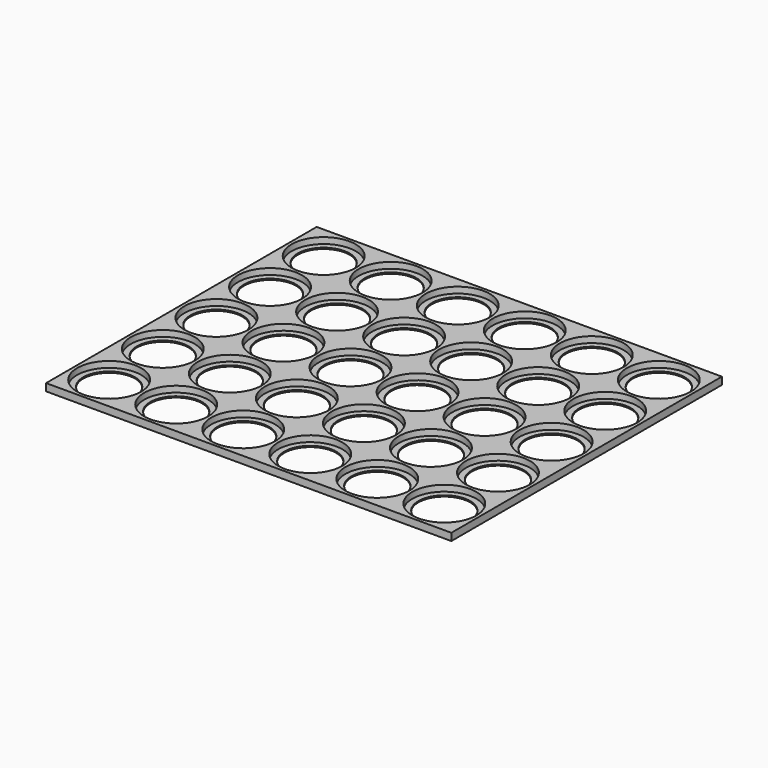
from build123d import *

# Parameters (mm, degrees)
F1_W      = 133
F1_H      = 111
F1_R      = 10.5
F2_DEPTH  = 2
F2_FACE_W = 133
F2_FACE_H = 111
F2_FACE_R = 10.5
F3_DEPTH  = 0.4
F4_D      = 17


# Not quite as in the source:
# - a feature of the source that left no trace in its solid (it failed there, or was rolled back) is left out


with BuildPart() as f2:
    # F1 (on Top) → F2 (new body)
    with BuildSketch(Plane.XY):
        with Locations((55, 44)):
            Rectangle(F1_W, F1_H)
        Circle(F1_R, mode=Mode.SUBTRACT)
        with Locations((22, 0)):
            Circle(F1_R, mode=Mode.SUBTRACT)
        with Locations((44, 0)):
            Circle(F1_R, mode=Mode.SUBTRACT)
        with Locations((0, 22)):
            Circle(F1_R, mode=Mode.SUBTRACT)
        with Locations((22, 22)):
            Circle(F1_R, mode=Mode.SUBTRACT)
        with Locations((44, 22)):
            Circle(F1_R, mode=Mode.SUBTRACT)
        with Locations((66, 0)):
            Circle(F1_R, mode=Mode.SUBTRACT)
        with Locations((88, 0)):
            Circle(F1_R, mode=Mode.SUBTRACT)
        with Locations((110, 0)):
            Circle(F1_R, mode=Mode.SUBTRACT)
        with Locations((66, 22)):
            Circle(F1_R, mode=Mode.SUBTRACT)
        with Locations((88, 22)):
            Circle(F1_R, mode=Mode.SUBTRACT)
        with Locations((110, 22)):
            Circle(F1_R, mode=Mode.SUBTRACT)
        with Locations((0, 44)):
            Circle(F1_R, mode=Mode.SUBTRACT)
        with Locations((0, 66)):
            Circle(F1_R, mode=Mode.SUBTRACT)
        with Locations((22, 44)):
            Circle(F1_R, mode=Mode.SUBTRACT)
        with Locations((44, 44)):
            Circle(F1_R, mode=Mode.SUBTRACT)
        with Locations((22, 66)):
            Circle(F1_R, mode=Mode.SUBTRACT)
        with Locations((44, 66)):
            Circle(F1_R, mode=Mode.SUBTRACT)
        with Locations((0, 88)):
            Circle(F1_R, mode=Mode.SUBTRACT)
        with Locations((22, 88)):
            Circle(F1_R, mode=Mode.SUBTRACT)
        with Locations((44, 88)):
            Circle(F1_R, mode=Mode.SUBTRACT)
        with Locations((66, 44)):
            Circle(F1_R, mode=Mode.SUBTRACT)
        with Locations((88, 44)):
            Circle(F1_R, mode=Mode.SUBTRACT)
        with Locations((66, 66)):
            Circle(F1_R, mode=Mode.SUBTRACT)
        with Locations((88, 66)):
            Circle(F1_R, mode=Mode.SUBTRACT)
        with Locations((110, 44)):
            Circle(F1_R, mode=Mode.SUBTRACT)
        with Locations((110, 66)):
            Circle(F1_R, mode=Mode.SUBTRACT)
        with Locations((66, 88)):
            Circle(F1_R, mode=Mode.SUBTRACT)
        with Locations((88, 88)):
            Circle(F1_R, mode=Mode.SUBTRACT)
        with Locations((110, 88)):
            Circle(F1_R, mode=Mode.SUBTRACT)
    extrude(amount=F2_DEPTH)

    # F2_face (on face) + F1 (on Top) → F3 (join)
    with BuildSketch(Plane(origin=(55, 44, 2), x_dir=(1, 0, 0), z_dir=(0, 0, 1))):
        Rectangle(F2_FACE_W, F2_FACE_H)
        with Locations((-55, -44)):
            Circle(F2_FACE_R, mode=Mode.SUBTRACT)
        with Locations((-33, -44)):
            Circle(F2_FACE_R, mode=Mode.SUBTRACT)
        with Locations((-11, -44)):
            Circle(F2_FACE_R, mode=Mode.SUBTRACT)
        with Locations((-55, -22)):
            Circle(F2_FACE_R, mode=Mode.SUBTRACT)
        with Locations((-33, -22)):
            Circle(F2_FACE_R, mode=Mode.SUBTRACT)
        with Locations((-11, -22)):
            Circle(F2_FACE_R, mode=Mode.SUBTRACT)
        with Locations((11, -44)):
            Circle(F2_FACE_R, mode=Mode.SUBTRACT)
        with Locations((33, -44)):
            Circle(F2_FACE_R, mode=Mode.SUBTRACT)
        with Locations((55, -44)):
            Circle(F2_FACE_R, mode=Mode.SUBTRACT)
        with Locations((11, -22)):
            Circle(F2_FACE_R, mode=Mode.SUBTRACT)
        with Locations((33, -22)):
            Circle(F2_FACE_R, mode=Mode.SUBTRACT)
        with Locations((55, -22)):
            Circle(F2_FACE_R, mode=Mode.SUBTRACT)
        with Locations((-55, 0)):
            Circle(F2_FACE_R, mode=Mode.SUBTRACT)
        with Locations((-55, 22)):
            Circle(F2_FACE_R, mode=Mode.SUBTRACT)
        with Locations((-33, 0)):
            Circle(F2_FACE_R, mode=Mode.SUBTRACT)
        with Locations((-11, 0)):
            Circle(F2_FACE_R, mode=Mode.SUBTRACT)
        with Locations((-33, 22)):
            Circle(F2_FACE_R, mode=Mode.SUBTRACT)
        with Locations((-11, 22)):
            Circle(F2_FACE_R, mode=Mode.SUBTRACT)
        with Locations((-55, 44)):
            Circle(F2_FACE_R, mode=Mode.SUBTRACT)
        with Locations((-33, 44)):
            Circle(F2_FACE_R, mode=Mode.SUBTRACT)
        with Locations((-11, 44)):
            Circle(F2_FACE_R, mode=Mode.SUBTRACT)
        with Locations((11, 0)):
            Circle(F2_FACE_R, mode=Mode.SUBTRACT)
        with Locations((33, 0)):
            Circle(F2_FACE_R, mode=Mode.SUBTRACT)
        with Locations((11, 22)):
            Circle(F2_FACE_R, mode=Mode.SUBTRACT)
        with Locations((33, 22)):
            Circle(F2_FACE_R, mode=Mode.SUBTRACT)
        with Locations((55, 0)):
            Circle(F2_FACE_R, mode=Mode.SUBTRACT)
        with Locations((55, 22)):
            Circle(F2_FACE_R, mode=Mode.SUBTRACT)
        with Locations((11, 44)):
            Circle(F2_FACE_R, mode=Mode.SUBTRACT)
        with Locations((33, 44)):
            Circle(F2_FACE_R, mode=Mode.SUBTRACT)
        with Locations((55, 44)):
            Circle(F2_FACE_R, mode=Mode.SUBTRACT)
    with BuildSketch(Plane.XY):
        with Locations((0, 88)):
            Circle(F1_R)
        with Locations((22, 88)):
            Circle(F1_R)
        with Locations((44, 88)):
            Circle(F1_R)
        with Locations((66, 88)):
            Circle(F1_R)
        with Locations((88, 88)):
            Circle(F1_R)
        with Locations((110, 88)):
            Circle(F1_R)
        with Locations((110, 66)):
            Circle(F1_R)
        with Locations((88, 66)):
            Circle(F1_R)
        with Locations((66, 66)):
            Circle(F1_R)
        with Locations((44, 66)):
            Circle(F1_R)
        with Locations((22, 66)):
            Circle(F1_R)
        with Locations((0, 66)):
            Circle(F1_R)
        with Locations((22, 44)):
            Circle(F1_R)
        with Locations((0, 44)):
            Circle(F1_R)
        with Locations((44, 44)):
            Circle(F1_R)
        with Locations((66, 44)):
            Circle(F1_R)
        with Locations((88, 44)):
            Circle(F1_R)
        with Locations((110, 44)):
            Circle(F1_R)
        with Locations((110, 22)):
            Circle(F1_R)
        with Locations((88, 22)):
            Circle(F1_R)
        with Locations((66, 22)):
            Circle(F1_R)
        with Locations((44, 22)):
            Circle(F1_R)
        with Locations((22, 22)):
            Circle(F1_R)
        with Locations((0, 22)):
            Circle(F1_R)
        Circle(F1_R)
        with Locations((22, 0)):
            Circle(F1_R)
        with Locations((44, 0)):
            Circle(F1_R)
        with Locations((66, 0)):
            Circle(F1_R)
        with Locations((88, 0)):
            Circle(F1_R)
        with Locations((110, 0)):
            Circle(F1_R)
    extrude(amount=F3_DEPTH)

    # F4 (through all)
    with Locations(Plane(origin=(0, 0, 0), x_dir=(1, 0, 0), z_dir=(0, 0, -1))):
        with Locations((0, -88), (22, -88), (44, -88), (66, -88), (88, -88), (110, -88), (110, -66), (88, -66), (66, -66), (44, -66), (22, -66), (0, -66), (0, -44), (22, -44), (44, -44), (66, -44), (88, -44), (110, -44), (110, -22), (88, -22), (66, -22), (44, -22), (22, -22), (0, -22), (110, 0), (88, 0), (66, 0), (44, 0), (22, 0), (0, 0)):
            Hole(F4_D / 2)


solid = f2.part
